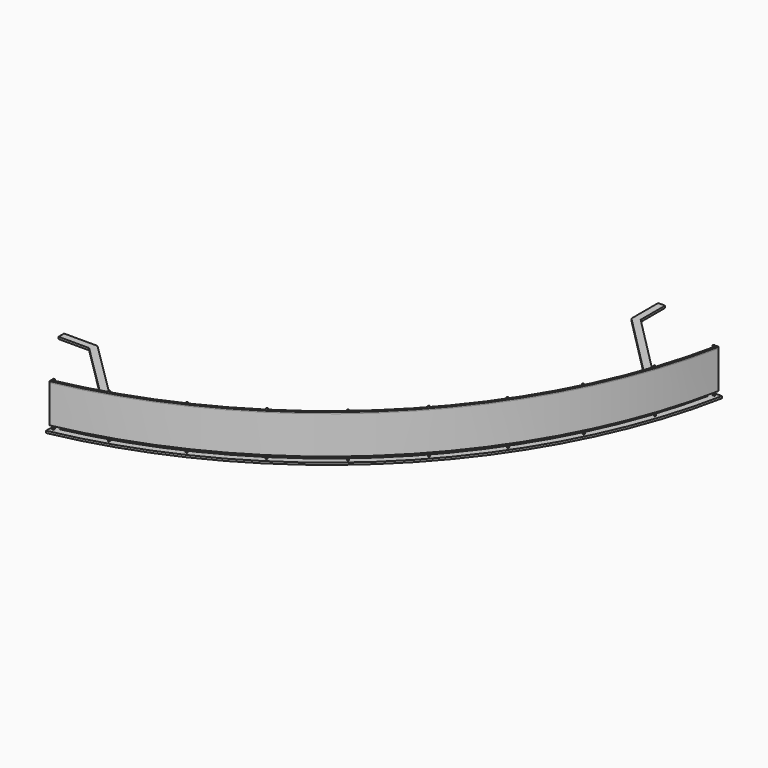
from build123d import *

# Parameters (mm, degrees)
F2_DEPTH  = 150
F3_W      = 150
F3_H      = 100
F3_W_2    = 100
F3_H_2    = 150
F4_DEPTH  = 3300
F7_DEPTH  = 3300
F9_ANGLE  = 90
F10_W     = 133
F10_H     = 2800
F11_ANGLE = 90
F12_W     = 6750
F12_H     = 3694.4781839848
F13_DEPTH = 34185.001
F14_W     = 6750
F14_H     = 4040.5442416668
F15_DEPTH = 34185.001


# Not quite as in the source:
# - a pattern or mirror of a feature is missing from the dataset's text; its kind, count and spacing are read off the source's solid


with BuildPart() as f2:
    # F1 (on Top) → F2 (new body)
    with BuildSketch(Plane.XY):
        with BuildLine():
            Line((6600, -28623.3583242364), (6600, -33623.3583242364))
            ThreePointArc((6600, -33623.3583242364), (24229.0138573571, -24229.0138573571), (33623.3583242364, -6600))
            Line((33623.3583242364, -6600), (28623.3583242364, -6600))
            Line((28623.3583242364, -6600), (24255.2923906681, -2200))
            Line((24255.2923906681, -2200), (24255.2923906681, 0))
            Line((24255.2923906681, 0), (23755.2923906681, 0))
            Line((23755.2923906681, 0), (23755.2923906681, -2406.040845923))
            Line((23755.2923906681, -2406.040845923), (28415.1839985056, -7100))
            Line((28415.1839985056, -7100), (33010.0776279002, -7100))
            ThreePointArc((33010.0776279002, -7100), (23875.4604667638, -23875.4604667638), (7100, -33010.0776279002))
            Line((7100, -33010.0776279002), (7100, -28415.1839985056))
            Line((7100, -28415.1839985056), (2406.040845923, -23755.2923906681))
            Line((2406.040845923, -23755.2923906681), (0, -23755.2923906681))
            Line((0, -23755.2923906681), (0, -24255.2923906681))
            Line((0, -24255.2923906681), (2200, -24255.2923906681))
            Line((2200, -24255.2923906681), (6600, -28623.3583242364))
        make_face()
    extrude(amount=F2_DEPTH)

    # F3 (on Top) → F4 (join)
    with BuildSketch(Plane.XY):
        with Locations((33215, -6800)):
            Rectangle(F3_W, F3_H)
        with Locations((6800, -33215)):
            Rectangle(F3_W_2, F3_H_2)
    extrude(amount=F4_DEPTH)

    # F6 (on Top) → F7 (join)
    with BuildSketch(Plane.XY):
        Polygon((32112.1251704395, -10754.1685888787), (32096.1772049746, -10801.5570093792), (32080.2292395097, -10848.9454298796), (32222.3945010112, -10896.7893262743), (32238.3424664761, -10849.4009057739), (32254.290431941, -10802.0124852734), align=None)
    f7 = extrude(amount=F7_DEPTH)

    # F7_copies: F7 across plane
    add(f7.mirror(Plane(origin=(0, 0, 0), x_dir=(-0.9241655206, 0.3819922651, 0), z_dir=(-0.3819922651, -0.9241655206, 0))))

    # F7_copies1: F7 across plane
    add(f7.mirror(Plane(origin=(0, 0, 0), x_dir=(-0.8963759304, 0.4432947005, 0), z_dir=(-0.4432947005, -0.8963759304, 0))))

    # F7_copies2: F7 across plane
    add(f7.mirror(Plane(origin=(0, 0, 0), x_dir=(-0.8645255332, 0.5025889001, 0), z_dir=(-0.5025889001, -0.8645255332, 0))))

    # F7_copies3: F7 across plane
    add(f7.mirror(Plane(origin=(0, 0, 0), x_dir=(-0.8287586193, 0.5596062464, 0), z_dir=(-0.5596062464, -0.8287586193, 0))))

    # F7_copies4: F7 across plane
    add(f7.mirror(Plane(origin=(0, 0, 0), x_dir=(-0.7892372217, 0.6140884365, 0), z_dir=(-0.6140884365, -0.7892372217, 0))))

    # F7_copies5: F7 across plane
    add(f7.mirror(Plane(origin=(0, 0, 0), x_dir=(-0.7461403823, 0.6657886526, 0), z_dir=(-0.6657886526, -0.7461403823, 0))))

    # F7_copies6: F7 across plane
    add(f7.mirror(Plane(origin=(0, 0, 0), x_dir=(0.6996633405, -0.7144726796, 0), z_dir=(-0.7144726796, -0.6996633405, 0))))


with BuildPart() as f9:
    # F8 (on Front) → F9 (revolve)
    with BuildSketch(Plane.XZ):
        Polygon((34185, 3300), (34035, 3300), (34035, 3200), (34041, 3200), (34041, 3294), (34179, 3294), (34179, 3200), (34185, 3200), align=None)
    revolve(axis=Axis((0, 0, 3739.7677898407), (0, 0, -1)), revolution_arc=F9_ANGLE)


with BuildPart() as f11:
    # F10 (on Front) → F11 (revolve)
    with BuildSketch(Plane.XZ):
        with Locations((34110, 1889)):
            Rectangle(F10_W, F10_H)
    revolve(axis=Axis((0, 0, 3739.7677898407), (0, 0, -1)), revolution_arc=F11_ANGLE)


with BuildPart() as f13_tool:
    # F12 (on Front) → F13 (new body, through all)
    with BuildSketch(Plane.XZ):
        with Locations((3375, 2133.2916468382)):
            Rectangle(F12_W, F12_H)
    extrude(amount=F13_DEPTH)


with BuildPart() as f9_1:
    add(f9.part)

    # F13: cut by f13_tool
    add(f13_tool.part, mode=Mode.SUBTRACT)


with BuildPart() as f11_1:
    add(f11.part)

    # F13: cut by f13_tool
    add(f13_tool.part, mode=Mode.SUBTRACT)


with BuildPart() as f15_tool:
    # F14 (on Right) → F15 (new body, through all)
    with BuildSketch(Plane.YZ):
        with Locations((-3375, 2345.6932455301)):
            Rectangle(F14_W, F14_H)
    extrude(amount=F15_DEPTH)


with BuildPart() as f9_2:
    add(f9_1.part)

    # F15: cut by f15_tool
    add(f15_tool.part, mode=Mode.SUBTRACT)


with BuildPart() as f11_2:
    add(f11_1.part)

    # F15: cut by f15_tool
    add(f15_tool.part, mode=Mode.SUBTRACT)


solid = Compound([f2.part, f9_2.part, f11_2.part])
